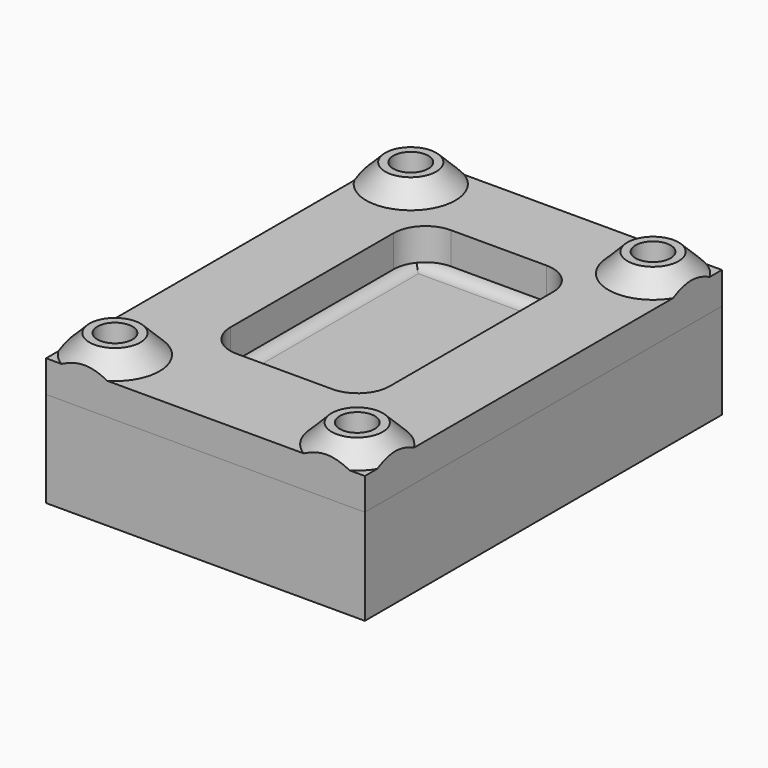
from build123d import *

# Parameters (mm, degrees)
F0_W     = 30
F0_H     = 50
F1_DEPTH = 15
F2_R     = 4.35
F2_R_2   = 2.75
F3_DEPTH = 8
F4_DEPTH = 3
F5_R     = 2
F6_W     = 50
F6_H     = 70
F6_R     = 4
F6_W_2   = 30
F6_H_2   = 50
F6_W_3   = 25
F6_H_3   = 45
F6_R_2   = 2.75
F7_DEPTH = 5
F8_DEPTH = 8
F9_DEPTH = 3
F11_R    = 5


# Not quite as in the source:
# - a fillet or chamfer that OpenCascade refuses, or shapes differently, is made with other operations: its cross-section is extruded or revolved along the edge and cut away or added


with BuildPart() as f1:
    # F0 (on Top) → F1 (new body)
    with BuildSketch(Plane.XY):
        with BuildLine():
            Line((19, 31.75), (19, 35))
            Line((19, 35), (-19, 35))
            Line((-19, 35), (-25, 35))
            Line((-25, 35), (-25, -29))
            Line((-25, -29), (-21.75, -29))
            ThreePointArc((-21.75, -29), (-19, -26.25), (-16.25, -29))
            ThreePointArc((-16.25, -29), (-17.0554563517, -30.9445436483), (-19, -31.75))
            Line((-19, -31.75), (-19, -35))
            Line((-19, -35), (19, -35))
            Line((19, -35), (19, -31.75))
            ThreePointArc((19, -31.75), (17.0554563517, -27.0554563517), (21.75, -29))
            Line((21.75, -29), (25, -29))
            Line((25, -29), (25, 29))
            Line((25, 29), (21.75, 29))
            ThreePointArc((21.75, 29), (17.0554563517, 27.0554563517), (19, 31.75))
        make_face()
        with BuildLine():
            ThreePointArc((-16.25, 29), (-20.9445436483, 27.0554563517), (-19, 31.75))
            ThreePointArc((-19, 31.75), (-17.0554563517, 30.9445436483), (-16.25, 29))
        make_face(mode=Mode.SUBTRACT)
        Rectangle(F0_W, F0_H, mode=Mode.SUBTRACT)
        with BuildLine():
            Line((25, 29), (25, 35))
            Line((25, 35), (19, 35))
            Line((19, 35), (19, 31.75))
            ThreePointArc((19, 31.75), (20.9445436483, 30.9445436483), (21.75, 29))
            Line((21.75, 29), (25, 29))
        make_face()
        with BuildLine():
            Line((25, -35), (25, -29))
            Line((25, -29), (21.75, -29))
            ThreePointArc((21.75, -29), (20.9445436483, -30.9445436483), (19, -31.75))
            Line((19, -31.75), (19, -35))
            Line((19, -35), (25, -35))
        make_face()
        with BuildLine():
            Line((-21.75, -29), (-25, -29))
            Line((-25, -29), (-25, -35))
            Line((-25, -35), (-19, -35))
            Line((-19, -35), (-19, -31.75))
            ThreePointArc((-19, -31.75), (-20.9445436483, -30.9445436483), (-21.75, -29))
        make_face()
        Rectangle(F0_W, F0_H)
    extrude(amount=-F1_DEPTH)

    # F2 (on face) → F3 (cut)
    with BuildSketch(Plane(origin=(0, 0, -15), x_dir=(1, 0, 0), z_dir=(0, 0, -1))):
        with Locations((-19, 29)):
            Circle(F2_R)
        with Locations((-19, 29)):
            Circle(F2_R_2, mode=Mode.SUBTRACT)
        with Locations((19, 29)):
            Circle(F2_R)
        with Locations((19, 29)):
            Circle(F2_R_2, mode=Mode.SUBTRACT)
        with Locations((19, -29)):
            Circle(F2_R)
        with Locations((19, -29)):
            Circle(F2_R_2, mode=Mode.SUBTRACT)
        with Locations((-19, -29)):
            Circle(F2_R)
        with Locations((-19, -29)):
            Circle(F2_R_2, mode=Mode.SUBTRACT)
    extrude(amount=-F3_DEPTH, mode=Mode.SUBTRACT)

    # F0 (on Top) → F4 (cut)
    with BuildSketch(Plane.XY):
        Rectangle(F0_W, F0_H)
    extrude(amount=-F4_DEPTH, mode=Mode.SUBTRACT)

    # F5
    f5_edges = [f1.edges().sort_by_distance(p)[0] for p in [
        (0, 25, -3),
        (15, 0, -3),
        (-15, 0, -3),
        (0, -25, -3),
    ]]
    fillet(f5_edges, radius=F5_R)


with BuildPart() as f7:
    # F6 (on face) → F7 (new body)
    with BuildSketch(Plane.XY):
        Rectangle(F6_W, F6_H)
        with Locations((-19, -29)):
            Circle(F6_R, mode=Mode.SUBTRACT)
        with Locations((19, -29)):
            Circle(F6_R, mode=Mode.SUBTRACT)
        with Locations((-19, 29)):
            Circle(F6_R, mode=Mode.SUBTRACT)
        Rectangle(F6_W_2, F6_H_2, mode=Mode.SUBTRACT)
        with Locations((19, 29)):
            Circle(F6_R, mode=Mode.SUBTRACT)
        Rectangle(F6_W_2, F6_H_2)
        Rectangle(F6_W_3, F6_H_3, mode=Mode.SUBTRACT)
        with Locations((19, -29)):
            Circle(F6_R)
        with Locations((19, -29)):
            Circle(F6_R_2, mode=Mode.SUBTRACT)
        with Locations((-19, -29)):
            Circle(F6_R)
        with Locations((-19, -29)):
            Circle(F6_R_2, mode=Mode.SUBTRACT)
        with Locations((19, 29)):
            Circle(F6_R)
        with Locations((19, 29)):
            Circle(F6_R_2, mode=Mode.SUBTRACT)
        with Locations((-19, 29)):
            Circle(F6_R)
        with Locations((-19, 29)):
            Circle(F6_R_2, mode=Mode.SUBTRACT)
    extrude(amount=F7_DEPTH)

    # F6 (on face) → F8 (join)
    with BuildSketch(Plane.XY):
        with Locations((19, 29)):
            Circle(F6_R)
        with Locations((19, 29)):
            Circle(F6_R_2, mode=Mode.SUBTRACT)
        with Locations((-19, 29)):
            Circle(F6_R)
        with Locations((-19, 29)):
            Circle(F6_R_2, mode=Mode.SUBTRACT)
        with Locations((-19, -29)):
            Circle(F6_R)
        with Locations((-19, -29)):
            Circle(F6_R_2, mode=Mode.SUBTRACT)
        with Locations((19, -29)):
            Circle(F6_R)
        with Locations((19, -29)):
            Circle(F6_R_2, mode=Mode.SUBTRACT)
    extrude(amount=F8_DEPTH)

    # F9 (add): a face of the model
    f9_faces = [f7.faces().sort_by_distance(p)[0] for p in [
        (0, -22.5, 2.5),
    ]]
    extrude(f9_faces, amount=F9_DEPTH)

    # F10: chamfer of 3 on 4 edges, made by hand


with BuildPart() as f10_tool2:
    # F10_s3 → F10_t4 (revolve)
    with BuildSketch(Plane.XZ.offset(-29)):
        Polygon((26, 5), (23, 8), (23, 5), align=None)
    revolve(axis=Axis((19, 29, 5), (0, 0, -1)))

    split(bisect_by=Plane.YZ.offset(25), keep=Keep.BOTTOM)

    split(bisect_by=Plane.XZ.offset(-35), keep=Keep.TOP)

    split(bisect_by=Plane.XY.offset(8), keep=Keep.BOTTOM)


with BuildPart() as f7_1:
    add(f7.part)

    # F10_t1: union F10_tool2
    add(f10_tool2.part)


with BuildPart() as f10_tool9:
    # F10_s10 → F10_t11 (revolve)
    with BuildSketch(Plane.XZ.offset(29)):
        Polygon((26, 5), (23, 8), (23, 5), align=None)
    revolve(axis=Axis((19, -29, 5), (0, 0, -1)))

    split(bisect_by=Plane.YZ.offset(25), keep=Keep.BOTTOM)

    split(bisect_by=Plane.XZ.offset(35), keep=Keep.BOTTOM)

    split(bisect_by=Plane.XY.offset(8), keep=Keep.BOTTOM)


with BuildPart() as f7_2:
    add(f7_1.part)

    # F10_t8: union F10_tool9
    add(f10_tool9.part)


with BuildPart() as f10_tool16:
    # F10_s17 → F10_t18 (revolve)
    with BuildSketch(Plane.XZ.offset(29)):
        Polygon((-12, 5), (-15, 8), (-15, 5), align=None)
    revolve(axis=Axis((-19, -29, 5), (0, 0, -1)))

    split(bisect_by=Plane.XZ.offset(35), keep=Keep.BOTTOM)

    split(bisect_by=Plane.YZ.offset(-25), keep=Keep.TOP)

    split(bisect_by=Plane.XY.offset(8), keep=Keep.BOTTOM)


with BuildPart() as f7_3:
    add(f7_2.part)

    # F10_t15: union F10_tool16
    add(f10_tool16.part)


with BuildPart() as f10_tool23:
    # F10_s24 → F10_t25 (revolve)
    with BuildSketch(Plane.XZ.offset(-29)):
        Polygon((-12, 5), (-15, 8), (-15, 5), align=None)
    revolve(axis=Axis((-19, 29, 5), (0, 0, -1)))

    split(bisect_by=Plane.XZ.offset(-35), keep=Keep.TOP)

    split(bisect_by=Plane.YZ.offset(-25), keep=Keep.TOP)

    split(bisect_by=Plane.XY.offset(8), keep=Keep.BOTTOM)


with BuildPart() as f7_4:
    add(f7_3.part)

    # F10_t22: union F10_tool23
    add(f10_tool23.part)

    # F11
    f11_edges = [f7_4.edges().sort_by_distance(p)[0] for p in [
        (-12.5, -19.5, 2.5),
        (12.5, -19.5, 2.5),
        (-12.5, 22.5, 2.5),
        (12.5, 22.5, 2.5),
    ]]
    fillet(f11_edges, radius=F11_R)


solid = Compound([f1.part, f7_4.part])
